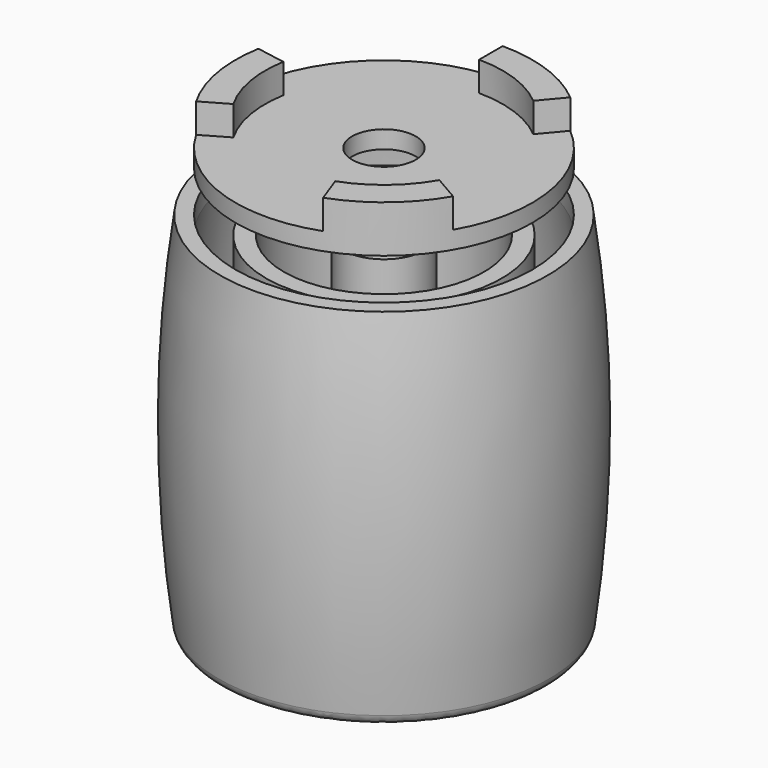
from build123d import *

# Parameters (mm, degrees)
F1_W     = 19.8026703335
F1_H     = 3
F4_R     = 2
F7_DEPTH = 5


# Not quite as in the source:
# - two fillets or chamfers of one size are made in one step
# - after a boolean that leaves OpenCascade's solid faulty, fix() repairs it


with BuildPart() as f2:
    # F0 (on Front) → F2 (revolve)
    with BuildSketch(Plane.XZ):
        with BuildLine():
            Line((-27.8249303423, 0), (0, 0))
            Line((0, 0), (0, 27.5))
            Line((0, 27.5), (-5.4, 27.5))
            Line((-5.4, 27.5), (-5.4, 59))
            Line((-5.4, 59), (-7, 59))
            Line((-7, 59), (-7, 3))
            Line((-7, 3), (-17, 3))
            Line((-17, 3), (-17, 59))
            Line((-17, 59), (-20, 59))
            Line((-20, 59), (-20, 3))
            Line((-20, 3), (-25.2026703335, 3))
            ThreePointArc((-25.2026703335, 3), (-27, 31), (-25.2026703335, 59))
            Line((-25.2026703335, 59), (-25.2026703335, 62))
            Line((-25.2026703335, 62), (-27.8249303423, 62))
            ThreePointArc((-27.8249303423, 62), (-30, 31), (-27.8249303423, 0))
        make_face()
    revolve(axis=Axis((0, 0, 13.75), (0, 0, -1)))

    # F4
    f4_edges = [f2.edges().sort_by_distance(p)[0] for p in [
        (5.4, 0, 27.5),
        (17, 0, 3),
        (25.20267, 0, 3),
        (20, 0, 3),
        (27.82493, 0, 0),
        (7, 0, 3),
    ]]
    fillet(f4_edges, radius=F4_R)


with BuildPart() as f3:
    # F1 (on Front) → F3 (revolve)
    with BuildSketch(Plane.XZ):
        with Locations((-15.3013351667, 70.5)):
            Rectangle(F1_W, F1_H)
    revolve(axis=Axis((0, 0, 13.75), (0, 0, -1)))

    # F6 (on face) → F7 (join)
    with BuildSketch(Plane.XY.offset(72)):
        with BuildLine():
            Line((0, 25.2026703335), (0, 20.2026703335))
            ThreePointArc((0, 20.2026703335), (6.909720203, 18.9843002326), (12.986026173, 15.4761433451))
            Line((12.986026173, 15.4761433451), (16.1999642214, 19.3063655607))
            ThreePointArc((16.1999642214, 19.3063655607), (8.6198209197, 23.6827633365), (0, 25.2026703335))
        make_face()
        with BuildLine():
            ThreePointArc((8.6198209197, -23.6827633365), (16.1999642214, -19.3063655607), (21.826152752, -12.6013351667))
            Line((21.826152752, -12.6013351667), (17.4960257331, -10.1013351667))
            ThreePointArc((17.4960257331, -10.1013351667), (12.986026173, -15.4761433451), (6.909720203, -18.9843002326))
            Line((6.909720203, -18.9843002326), (8.6198209197, -23.6827633365))
        make_face()
        with BuildLine():
            Line((-19.895746376, 3.5081568874), (-24.819785141, 4.3763977758))
            ThreePointArc((-24.819785141, 4.3763977758), (-24.819785141, -4.3763977758), (-21.826152752, -12.6013351667))
            Line((-21.826152752, -12.6013351667), (-17.4960257331, -10.1013351667))
            ThreePointArc((-17.4960257331, -10.1013351667), (-19.895746376, -3.5081568874), (-19.895746376, 3.5081568874))
        make_face()
    extrude(amount=F7_DEPTH)

    add(f3.part.fix(), mode=Mode.REPLACE)


solid = Compound([f2.part, f3.part])
